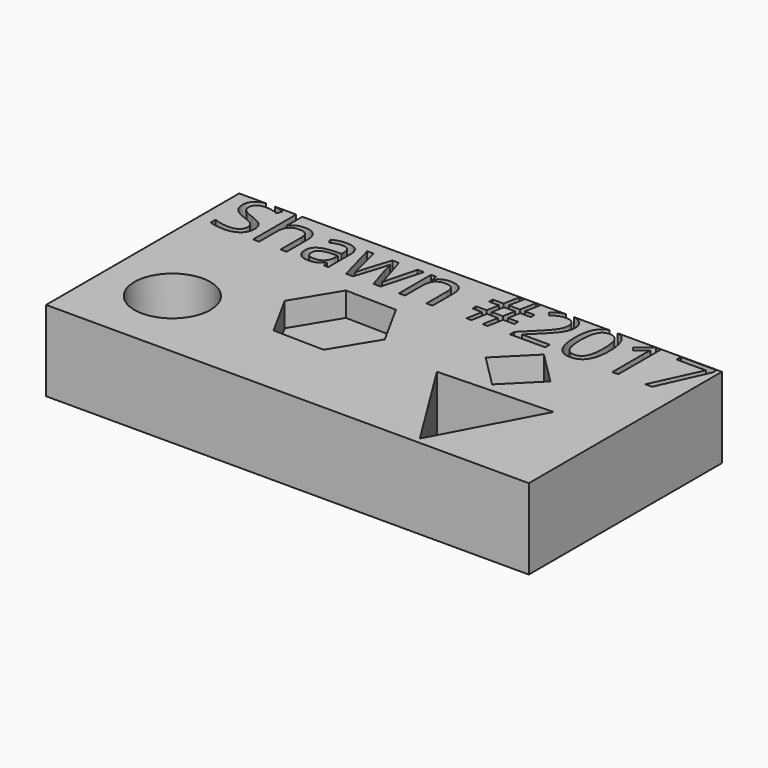
from build123d import *

# Parameters (mm, degrees)
F0_W         = 76.2
F0_H         = 38.1
F1_DEPTH     = 12.7
F3_DEPTH     = 3.81
F4_R         = 5.9936379925
F5_DEPTH     = 12.7
F7_DEPTH     = 12.7
F8_TEXT_SIZE = 11.8254504529
F9_DEPTH     = 12.7
F11_DEPTH    = 6.35


# Not quite as in the source:
# - Text() gives the source's letters only with a copy of the font that has no kerning and outlines rounded to 1/6400 em; it was checked with that copy


with BuildPart() as f1:
    # F0 (on Top) → F1 (new body)
    with BuildSketch(Plane.XY):
        Rectangle(F0_W, F0_H)
    extrude(amount=F1_DEPTH)

    # F2 (on face) → F3 (cut)
    with BuildSketch(Plane.XY.offset(12.7)):
        Polygon((-15.8041413099, 0.1667244069), (-11.9326584816, -6.8723293662), (-3.9009176812, -7.0390537732), (0.2593402908, -0.1667244069), (-3.6121425376, 6.8723293662), (-11.6438833379, 7.0390537732), align=None)
    extrude(amount=-F3_DEPTH, mode=Mode.SUBTRACT)

    # F4 (on face) → F5 (cut)
    with BuildSketch(Plane.XY.offset(12.7)):
        with Locations((-27.4320002645, -7.4676000513)):
            Circle(F4_R)
    extrude(amount=-F5_DEPTH, mode=Mode.SUBTRACT)

    # F6 (on face) → F7 (cut)
    with BuildSketch(Plane.XY.offset(12.7)):
        Polygon((20.1605676273, -18.1297336647), (28.6074311873, -2.2918663046), (10.6680039316, -2.8956015594), align=None)
    extrude(amount=-F7_DEPTH, mode=Mode.SUBTRACT)

    # F8 (on face) → F9 (cut)
    with BuildSketch(Plane.XY.offset(12.7)):
        with Locations((-36.6017400564, 10.5356756739)):
            Text('Shawn #2017', F8_TEXT_SIZE, font='Open Sans', text_align=(TextAlign.LEFT, TextAlign.BOTTOM))
    extrude(amount=-F9_DEPTH, mode=Mode.SUBTRACT)

    # F10 (on face) → F11 (cut)
    with BuildSketch(Plane.XY.offset(12.7)):
        Polygon((18.0935468525, -1.2842018623), (23.2008583844, 3.8231096696), (18.0935468525, 8.9304212015), (12.9862353206, 3.8231096696), align=None)
    extrude(amount=-F11_DEPTH, mode=Mode.SUBTRACT)


solid = f1.part
